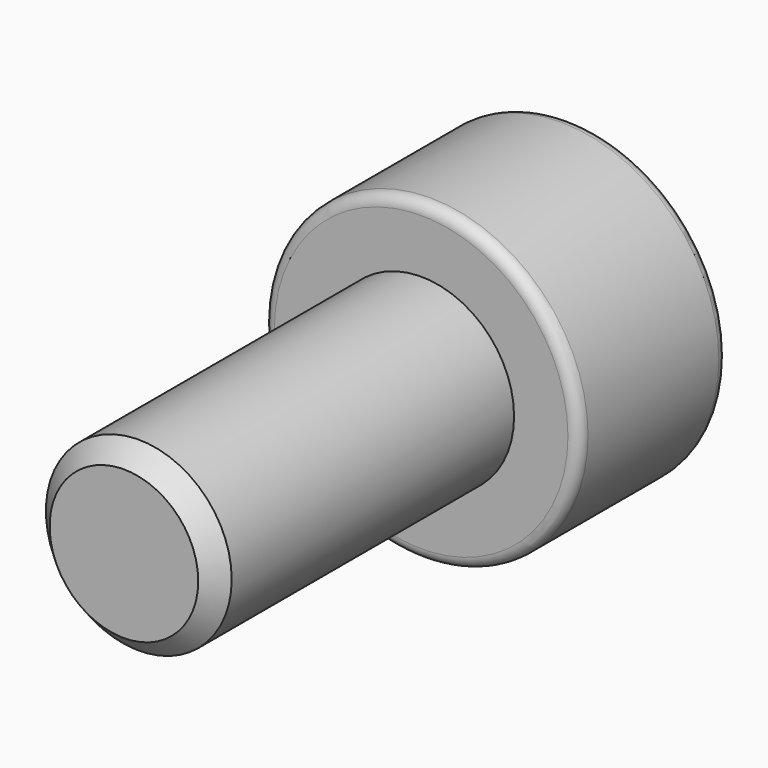
from build123d import *

# Parameters (mm, degrees)
F0_R     = 2.5
F1_DEPTH = 10
F2_SIZE  = 0.5
F3_R     = 4.25
F3_R_2   = 2.5
F4_DEPTH = 5
F6_DEPTH = 4
F7_R     = 0.3


with BuildPart() as f1:
    # F0 (on Front) → F1 (new body)
    with BuildSketch(Plane.XZ):
        Circle(F0_R)
    extrude(amount=F1_DEPTH)

    # F2
    f2_edges = [f1.edges().sort_by_distance(p)[0] for p in [
        (-2.5, -10, 0),
    ]]
    chamfer(f2_edges, length=F2_SIZE)

    # F3 (on face) → F4 (join)
    with BuildSketch(Plane(origin=(0, 0, 0), x_dir=(-1, 0, 0), z_dir=(0, 1, 0))):
        Circle(F3_R)
        Circle(F3_R_2, mode=Mode.SUBTRACT)
        Circle(F3_R_2)
    extrude(amount=F4_DEPTH)

    # F5 (on face) → F6 (cut)
    with BuildSketch(Plane(origin=(0, 5, 0), x_dir=(-1, 0, 0), z_dir=(0, 1, 0))):
        Polygon((-0.2009555222, 2.3006412609), (-2.092891538, 0.9762880432), (-1.8919360159, -1.3243532177), (0.2009555222, -2.3006412609), (2.092891538, -0.9762880432), (1.8919360159, 1.3243532177), align=None)
    extrude(amount=-F6_DEPTH, mode=Mode.SUBTRACT)

    # F7
    f7_edges = [f1.edges().sort_by_distance(p)[0] for p in [
        (4.25, 5, 0),
        (4.25, 0, 0),
        (1.146924, 5, 1.638465),
        (-0.84549, 5, 1.812497),
        (1.992414, 5, -0.174033),
        (0.84549, 5, -1.812497),
        (-1.146924, 5, -1.638465),
        (-1.992414, 5, 0.174033),
    ]]
    fillet(f7_edges, radius=F7_R)


solid = f1.part
